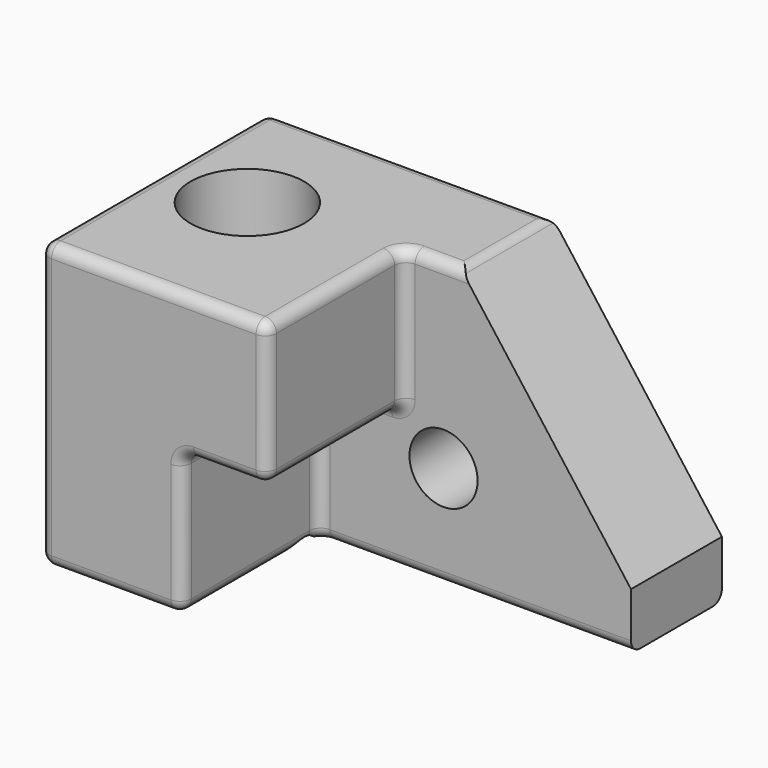
from build123d import *

# Parameters (mm, degrees)
F0_W     = 203.2
F0_H     = 127
F1_DEPTH = 127
F3_DEPTH = 76.2
F4_SIZE2 = 101.6
F4_SIZE  = 76.2
F5_R     = 5.08
F6_R     = 15.24
F7_DEPTH = 50.8
F8_R     = 25.4
F9_DEPTH = 127


with BuildPart() as f1:
    # F0 (on Front) → F1 (new body)
    with BuildSketch(Plane.XZ):
        with Locations((0.6489251732, -1.8226355314)):
            Rectangle(F0_W, F0_H)
    extrude(amount=F1_DEPTH)

    # F2 (on face) → F3 (cut)
    with BuildSketch(Plane.XZ.offset(127)):
        Polygon((102.2489251732, 61.6773644686), (0.6489251732, 61.6773644686), (0.6489251732, -1.8226355314), (-37.4510748268, -1.8226355314), (-37.4510748268, -65.3226355314), (102.2489251732, -65.3226355314), align=None)
    extrude(amount=-F3_DEPTH, mode=Mode.SUBTRACT)

    # F4
    f4_edges = [f1.edges().sort_by_distance(p)[0] for p in [
        (102.248925, -25.4, 61.677364),
    ]]
    f4_side = f1.faces().sort_by_distance((-21.122503, -52.614286, 61.677364))[0]
    chamfer(f4_edges, length=F4_SIZE, length2=F4_SIZE2, reference=f4_side)

    # F5
    f5_edges = [f1.edges().sort_by_distance(p)[0] for p in [
        (-50.151075, -127, 61.677364),
        (-37.451075, 0, 61.677364),
        (26.048925, -25.4, 61.677364),
        (-100.951075, -63.5, 61.677364),
        (13.348925, -50.8, 61.677364),
        (0.648925, -88.9, 61.677364),
        (0.648925, -127, 29.927364),
        (0.648925, -88.9, -1.822636),
        (0.648925, -50.8, 29.927364),
        (-37.451075, -88.9, -1.822636),
        (-37.451075, -88.9, -65.322636),
        (-37.451075, -127, -33.572636),
        (-37.451075, -50.8, -33.572636),
        (-69.201075, -127, -65.322636),
        (-100.951075, -63.5, -65.322636),
        (-100.951075, 0, -1.822636),
        (-100.951075, -127, -1.822636),
        (0.648925, 0, -65.322636),
        (32.398925, -50.8, -65.322636),
        (-18.401075, -50.8, -1.822636),
        (-18.401075, -127, -1.822636),
    ]]
    fillet(f5_edges, radius=F5_R)

    # F6 (on face) → F7 (cut, through all)
    with BuildSketch(Plane.XZ.offset(50.8)):
        with Locations((18.4289251732, -19.6026355314)):
            Circle(F6_R)
    extrude(amount=-F7_DEPTH, mode=Mode.SUBTRACT)

    # F8 (on face) → F9 (cut, through all)
    with BuildSketch(Plane.XY.offset(61.6773644686)):
        with Locations((-63.0807951093, -58.5683807731)):
            Circle(F8_R)
    extrude(amount=-F9_DEPTH, mode=Mode.SUBTRACT)


solid = f1.part
